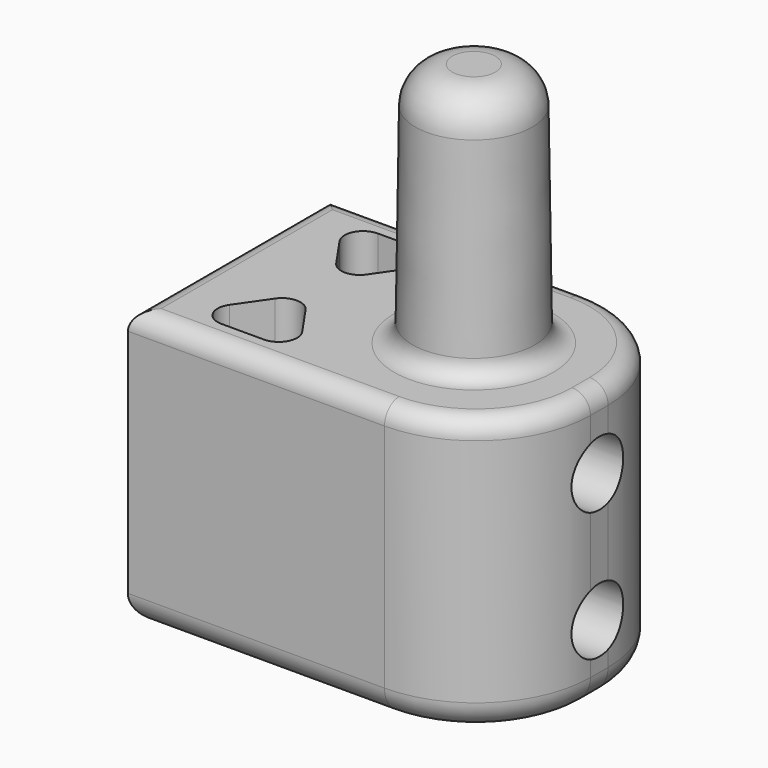
from build123d import *

# Parameters (mm, degrees)
F0_W         = 34.544
F0_H         = 34.544
F1_DEPTH     = 38.1
F3_R         = 15.748
F4_R         = 2.286
F5_DEPTH     = 34.545
F6_R         = 4.445
F7_DEPTH     = 27.94
F8_S5_R      = 4.445
F8_T6_DEPTH  = 8
F8_S11_R     = 4.445
F8_T12_DEPTH = 8
F9_DEPTH     = 16.51
F2_R         = 8.4455
F10_DEPTH    = 33.782
F10_TAPER    = 0.8
F11_R        = 2.54
F12_R        = 3.81
F13_R        = 5.08
F15_DEPTH    = 38.101


# Not quite as in the source:
# - a fillet or chamfer that OpenCascade refuses, or shapes differently, is made with other operations: its cross-section is extruded or revolved along the edge and cut away or added


with BuildPart() as f1:
    # F0 (on Top) → F1 (new body)
    with BuildSketch(Plane.XY):
        with Locations((17.272, -17.272)):
            Rectangle(F0_W, F0_H)
    extrude(amount=F1_DEPTH)

    # F3
    f3_edges = [f1.edges().sort_by_distance(p)[0] for p in [
        (34.544, -34.544, 19.05),
        (34.544, 0, 19.05),
    ]]
    fillet(f3_edges, radius=F3_R)

    # F4 (on face) → F5 (cut, through all)
    with BuildSketch(Plane(origin=(0, 0, 0), x_dir=(0, -1, 0), z_dir=(-1, 0, 0))):
        with Locations((17.272, 10.16)):
            Circle(F4_R)
        with Locations((17.272, 27.94)):
            Circle(F4_R)
    extrude(amount=-F5_DEPTH, mode=Mode.SUBTRACT)

    # F6 (on face) → F7 (cut)
    with BuildSketch(Plane.YZ.offset(34.544)):
        with Locations((-17.272, 27.94)):
            Circle(F6_R)
        with Locations((-17.272, 10.16)):
            Circle(F6_R)
    extrude(amount=-F7_DEPTH, mode=Mode.SUBTRACT)

    # F8: chamfer of 2.54 on 2 edges, made by hand


with BuildPart() as f8_tool2:
    # F8_s3 → F8_t4 (revolve)
    with BuildSketch(Plane.XY.offset(27.94)):
        Polygon((4.064, -19.558), (6.604, -22.098), (6.604, -19.558), align=None)
    revolve(axis=Axis((6.604, -17.272, 27.94), (-1, 0, 0)))

    # F8_s5 → F8_t6 (intersect, symmetric)
    with BuildSketch(Plane.YZ.offset(5.3)):
        with Locations((-17.272, 27.94)):
            Circle(F8_S5_R)
    extrude(amount=F8_T6_DEPTH, both=True, mode=Mode.INTERSECT)


with BuildPart() as f1_1:
    add(f1.part)

    # F8_t1: cut F8_tool2
    add(f8_tool2.part, mode=Mode.SUBTRACT)


with BuildPart() as f8_tool8:
    # F8_s9 → F8_t10 (revolve)
    with BuildSketch(Plane.XY.offset(10.16)):
        Polygon((4.064, -19.558), (6.604, -22.098), (6.604, -19.558), align=None)
    revolve(axis=Axis((6.604, -17.272, 10.16), (-1, 0, 0)))

    # F8_s11 → F8_t12 (intersect, symmetric)
    with BuildSketch(Plane.YZ.offset(5.3)):
        with Locations((-17.272, 10.16)):
            Circle(F8_S11_R)
    extrude(amount=F8_T12_DEPTH, both=True, mode=Mode.INTERSECT)


with BuildPart() as f1_2:
    add(f1_1.part)

    # F8_t7: cut F8_tool8
    add(f8_tool8.part, mode=Mode.SUBTRACT)

    # F9 (add): a face of the model
    f9_faces = [f1_2.faces().sort_by_distance(p)[0] for p in [
        (0, -17.272, 19.05),
    ]]
    extrude(f9_faces, amount=F9_DEPTH)

    # F2 (on face) → F10 (join)
    with BuildSketch(Plane.XY.offset(38.1)):
        with Locations((17.272, -17.272)):
            Circle(F2_R)
    extrude(amount=F10_DEPTH, taper=F10_TAPER)

    # F11
    f11_edges = [f1_2.edges().sort_by_distance(p)[0] for p in [
        (1.143, 0, 38.1),
        (-16.51, -17.272, 38.1),
        (29.931518, -4.612482, 38.1),
        (1.143, -34.544, 38.1),
        (34.544, -17.272, 38.1),
        (29.931518, -29.931518, 38.1),
        (8.8265, -17.272, 38.1),
    ]]
    fillet(f11_edges, radius=F11_R)

    # F12
    f12_edges = [f1_2.edges().sort_by_distance(p)[0] for p in [
        (1.143, 0, 0),
        (-16.51, -17.272, 0),
        (1.143, -34.544, 0),
        (29.931518, -29.931518, 0),
        (34.544, -17.272, 0),
        (29.931518, -4.612482, 0),
    ]]
    fillet(f12_edges, radius=F12_R)

    # F13
    f13_edges = [f1_2.edges().sort_by_distance(p)[0] for p in [
        (9.298216, -17.272, 71.882),
    ]]
    fillet(f13_edges, radius=F13_R)

    # F14 (on face) → F15 (cut, through all)
    with BuildSketch(Plane.XY.offset(38.1)):
        with BuildLine():
            ThreePointArc((-6.6983271655, -3.81), (-8.9482084501, -5.1711725294), (-8.7866908377, -7.7957998383))
            Line((-8.7866908377, -7.7957998383), (-5.8592190016, -12.0243421801))
            ThreePointArc((-5.8592190016, -12.0243421801), (-3.7708553294, -13.1185423418), (-1.6824916571, -12.0243421801))
            Line((-1.6824916571, -12.0243421801), (1.244980179, -7.7957998383))
            ThreePointArc((1.244980179, -7.7957998383), (1.4064977914, -5.1711725294), (-0.8433834932, -3.81))
            Line((-0.8433834932, -3.81), (-6.6983271655, -3.81))
        make_face()
        with BuildLine():
            ThreePointArc((-1.6824916571, -22.5196578199), (-3.7708553294, -21.4254576582), (-5.8592190016, -22.5196578199))
            Line((-5.8592190016, -22.5196578199), (-8.7866908377, -26.7482001617))
            ThreePointArc((-8.7866908377, -26.7482001617), (-8.9482084501, -29.3728274706), (-6.6983271655, -30.734))
            Line((-6.6983271655, -30.734), (-0.8433834932, -30.734))
            ThreePointArc((-0.8433834932, -30.734), (1.4064977914, -29.3728274706), (1.244980179, -26.7482001617))
            Line((1.244980179, -26.7482001617), (-1.6824916571, -22.5196578199))
        make_face()
    extrude(amount=-F15_DEPTH, mode=Mode.SUBTRACT)


solid = f1_2.part
